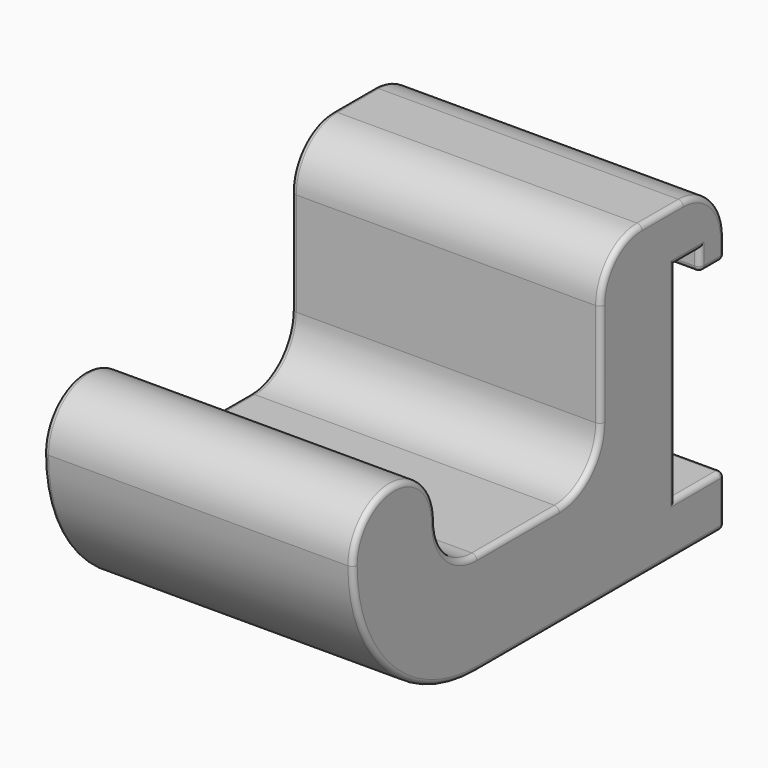
from build123d import *

# Parameters (mm, degrees)
F0_W         = 30
F0_H         = 30
F1_DEPTH     = 15
F3_DEPTH     = 30.001
F5_DEPTH     = 30
F6_R         = 5
F7_R         = 0.5
F8_T1_DEPTH  = 29
F8_S5_W      = 0.5
F8_S5_H      = 0.5
F8_T6_DEPTH  = 0.5
F8_S11_W     = 0.5
F8_S11_H     = 0.5
F8_T12_DEPTH = 0.5
F8_S17_W     = 0.5
F8_S17_H     = 0.5
F8_T18_DEPTH = 0.5
F8_S23_W     = 0.5
F8_S23_H     = 0.5
F8_T24_DEPTH = 0.5
F8_S29_W     = 0.5
F8_S29_H     = 0.5
F8_T30_DEPTH = 0.5
F8_S35_W     = 0.5
F8_S35_H     = 0.5
F8_T36_DEPTH = 0.5
F8_S41_W     = 0.5
F8_S41_H     = 0.5
F8_T42_DEPTH = 0.5
F8_S47_W     = 0.5
F8_S47_H     = 0.5
F8_T48_DEPTH = 0.5


# Not quite as in the source:
# - a fillet or chamfer that OpenCascade refuses, or shapes differently, is made with other operations: its cross-section is extruded or revolved along the edge and cut away or added


with BuildPart() as f1:
    # F0 (on Front) → F1 (new body)
    with BuildSketch(Plane.XZ):
        with Locations((15, 15)):
            Rectangle(F0_W, F0_H)
    extrude(amount=F1_DEPTH)

    # F2 (on face) → F3 (cut, through all)
    with BuildSketch(Plane.YZ.offset(30)):
        Polygon((-6, 5), (0, 5), (0, 23), (-3, 23), (-3, 25), (-6, 25), align=None)
    extrude(amount=-F3_DEPTH, mode=Mode.SUBTRACT)

    # F4 (on face) → F5 (join, through all)
    with BuildSketch(Plane.YZ.offset(30)):
        with BuildLine():
            Line((-30, 0), (-15, 0))
            Line((-15, 0), (-15, 10))
            Line((-15, 10), (-30, 10))
            ThreePointArc((-30, 10), (-33.5355339059, 11.4644660941), (-35, 15))
            ThreePointArc((-35, 15), (-40, 20), (-45, 15))
            ThreePointArc((-45, 15), (-40.6066017178, 4.3933982822), (-30, 0))
        make_face()
    extrude(amount=-F5_DEPTH)

    # F6
    f6_edges = [f1.edges().sort_by_distance(p)[0] for p in [
        (15, -15, 10),
        (15, -15, 30),
        (15, 0, 30),
    ]]
    fillet(f6_edges, radius=F6_R)

    # F7
    f7_edges = [f1.edges().sort_by_distance(p)[0] for p in [
        (30, -25, 10),
        (30, -16.464466, 11.464466),
        (30, -33.535534, 11.464466),
        (30, -15, 20),
        (30, -40, 20),
        (30, -13.535534, 28.535534),
        (30, -40.606602, 4.393398),
        (30, -7.5, 30),
        (30, -15, 0),
        (30, -1.464466, 28.535534),
        (30, 0, 2.5),
        (30, 0, 24),
        (30, -3, 5),
        (30, -1.5, 23),
        (30, -6, 15),
        (30, -3, 24),
        (30, -4.5, 25),
        (0, 0, 24),
        (0, -1.464466, 28.535534),
        (0, -1.5, 23),
        (0, -7.5, 30),
        (0, -3, 24),
        (0, -13.535534, 28.535534),
        (0, -4.5, 25),
        (0, -15, 20),
        (0, -6, 15),
        (0, -16.464466, 11.464466),
        (0, -3, 5),
        (0, -25, 10),
        (0, 0, 2.5),
        (0, -33.535534, 11.464466),
        (0, -15, 0),
        (0, -40, 20),
        (0, -40.606602, 4.393398),
    ]]
    fillet(f7_edges, radius=F7_R)

    # F8: fillet of radius 0.5 on 4 edges, made by hand

    # F8_s2 → F8_t1 (cut)
    with BuildSketch(Plane.YZ.offset(0.5)):
        with BuildLine():
            ThreePointArc((0, 4.5), (-0.1464466094, 4.8535533906), (-0.5, 5))
            Line((-0.5, 5), (0, 5))
            Line((0, 5), (0, 4.5))
        make_face()
        with BuildLine():
            ThreePointArc((-0.5, 0), (-0.1464466094, 0.1464466094), (0, 0.5))
            Line((0, 0.5), (0, 0))
            Line((0, 0), (-0.5, 0))
        make_face()
        with BuildLine():
            ThreePointArc((-0.5, 23), (-0.1464466094, 23.1464466094), (0, 23.5))
            Line((0, 23.5), (0, 23))
            Line((0, 23), (-0.5, 23))
        make_face()
        with BuildLine():
            ThreePointArc((-3, 23.5), (-2.8535533906, 23.1464466094), (-2.5, 23))
            Line((-2.5, 23), (-3, 23))
            Line((-3, 23), (-3, 23.5))
        make_face()
    extrude(amount=F8_T1_DEPTH, mode=Mode.SUBTRACT)


with BuildPart() as f8_tool4:
    # F8_s5 → F8_t6 (new body)
    with BuildSketch(Plane.XZ.offset(2.5)):
        with Locations((29.75, 23.25)):
            Rectangle(F8_S5_W, F8_S5_H)
    extrude(amount=F8_T6_DEPTH)

    # F8_s7 → F8_t8 (revolve, cut)
    with BuildSketch(Plane(origin=(29.5, -2.5, 23.5), x_dir=(-0.7071067812, 0, 0.7071067812), z_dir=(0.7071067812, 0, 0.7071067812))):
        with BuildLine():
            ThreePointArc((0, -0.5), (0.5, 0), (0, 0.5))
            Line((0, 0.5), (0, -0.5))
        make_face()
    revolve(axis=Axis((29.5, -2.5, 23.5), (0, -1, 0)), mode=Mode.SUBTRACT)


with BuildPart() as f1_1:
    add(f1.part)

    # F8_t3: cut F8_tool4
    add(f8_tool4.part, mode=Mode.SUBTRACT)


with BuildPart() as f8_tool10:
    # F8_s11 → F8_t12 (new body)
    with BuildSketch(Plane.XZ.offset(2.5)):
        with Locations((0.25, 23.25)):
            Rectangle(F8_S11_W, F8_S11_H)
    extrude(amount=F8_T12_DEPTH)

    # F8_s13 → F8_t14 (revolve, cut)
    with BuildSketch(Plane(origin=(0.5, -2.5, 23.5), x_dir=(0.7071067812, 0, 0.7071067812), z_dir=(0.7071067812, 0, -0.7071067812))):
        with BuildLine():
            ThreePointArc((0, -0.5), (0.5, 0), (0, 0.5))
            Line((0, 0.5), (0, -0.5))
        make_face()
    revolve(axis=Axis((0.5, -2.5, 23.5), (0, -1, 0)), mode=Mode.SUBTRACT)


with BuildPart() as f1_2:
    add(f1_1.part)

    # F8_t9: cut F8_tool10
    add(f8_tool10.part, mode=Mode.SUBTRACT)


with BuildPart() as f8_tool16:
    # F8_s17 → F8_t18 (new body)
    with BuildSketch(Plane.XY.offset(23.5)):
        with Locations((29.75, -0.25)):
            Rectangle(F8_S17_W, F8_S17_H)
    extrude(amount=-F8_T18_DEPTH)

    # F8_s19 → F8_t20 (revolve, cut)
    with BuildSketch(Plane(origin=(29.5, -0.5, 23.5), x_dir=(-0.7071067812, -0.7071067812, 0), z_dir=(0.7071067812, -0.7071067812, 0))):
        with BuildLine():
            ThreePointArc((0, -0.5), (0.5, 0), (0, 0.5))
            Line((0, 0.5), (0, -0.5))
        make_face()
    revolve(axis=Axis((29.5, -0.5, 23.5), (0, 0, -1)), mode=Mode.SUBTRACT)


with BuildPart() as f1_3:
    add(f1_2.part)

    # F8_t15: cut F8_tool16
    add(f8_tool16.part, mode=Mode.SUBTRACT)


with BuildPart() as f8_tool22:
    # F8_s23 → F8_t24 (new body)
    with BuildSketch(Plane.XY.offset(23.5)):
        with Locations((0.25, -0.25)):
            Rectangle(F8_S23_W, F8_S23_H)
    extrude(amount=-F8_T24_DEPTH)

    # F8_s25 → F8_t26 (revolve, cut)
    with BuildSketch(Plane(origin=(0.5, -0.5, 23.5), x_dir=(0.7071067812, -0.7071067812, 0), z_dir=(0.7071067812, 0.7071067812, 0))):
        with BuildLine():
            ThreePointArc((0, -0.5), (0.5, 0), (0, 0.5))
            Line((0, 0.5), (0, -0.5))
        make_face()
    revolve(axis=Axis((0.5, -0.5, 23.5), (0, 0, -1)), mode=Mode.SUBTRACT)


with BuildPart() as f1_4:
    add(f1_3.part)

    # F8_t21: cut F8_tool22
    add(f8_tool22.part, mode=Mode.SUBTRACT)


with BuildPart() as f8_tool28:
    # F8_s29 → F8_t30 (new body)
    with BuildSketch(Plane.XY.offset(0.5)):
        with Locations((0.25, -0.25)):
            Rectangle(F8_S29_W, F8_S29_H)
    extrude(amount=-F8_T30_DEPTH)

    # F8_s31 → F8_t32 (revolve, cut)
    with BuildSketch(Plane(origin=(0.5, -0.5, 0.5), x_dir=(0.7071067812, -0.7071067812, 0), z_dir=(0.7071067812, 0.7071067812, 0))):
        with BuildLine():
            ThreePointArc((0, -0.5), (0.5, 0), (0, 0.5))
            Line((0, 0.5), (0, -0.5))
        make_face()
    revolve(axis=Axis((0.5, -0.5, 0.5), (0, 0, -1)), mode=Mode.SUBTRACT)


with BuildPart() as f1_5:
    add(f1_4.part)

    # F8_t27: cut F8_tool28
    add(f8_tool28.part, mode=Mode.SUBTRACT)


with BuildPart() as f8_tool34:
    # F8_s35 → F8_t36 (new body)
    with BuildSketch(Plane.XY.offset(0.5)):
        with Locations((29.75, -0.25)):
            Rectangle(F8_S35_W, F8_S35_H)
    extrude(amount=-F8_T36_DEPTH)

    # F8_s37 → F8_t38 (revolve, cut)
    with BuildSketch(Plane(origin=(29.5, -0.5, 0.5), x_dir=(-0.7071067812, -0.7071067812, 0), z_dir=(0.7071067812, -0.7071067812, 0))):
        with BuildLine():
            ThreePointArc((0, -0.5), (0.5, 0), (0, 0.5))
            Line((0, 0.5), (0, -0.5))
        make_face()
    revolve(axis=Axis((29.5, -0.5, 0.5), (0, 0, -1)), mode=Mode.SUBTRACT)


with BuildPart() as f1_6:
    add(f1_5.part)

    # F8_t33: cut F8_tool34
    add(f8_tool34.part, mode=Mode.SUBTRACT)


with BuildPart() as f8_tool40:
    # F8_s41 → F8_t42 (new body)
    with BuildSketch(Plane.XZ.offset(0.5)):
        with Locations((29.75, 4.75)):
            Rectangle(F8_S41_W, F8_S41_H)
    extrude(amount=-F8_T42_DEPTH)

    # F8_s43 → F8_t44 (revolve, cut)
    with BuildSketch(Plane(origin=(29.5, -0.5, 4.5), x_dir=(-0.7071067812, 0, -0.7071067812), z_dir=(0.7071067812, 0, -0.7071067812))):
        with BuildLine():
            ThreePointArc((0, -0.5), (0.5, 0), (0, 0.5))
            Line((0, 0.5), (0, -0.5))
        make_face()
    revolve(axis=Axis((29.5, -0.5, 4.5), (0, 1, 0)), mode=Mode.SUBTRACT)


with BuildPart() as f1_7:
    add(f1_6.part)

    # F8_t39: cut F8_tool40
    add(f8_tool40.part, mode=Mode.SUBTRACT)


with BuildPart() as f8_tool46:
    # F8_s47 → F8_t48 (new body)
    with BuildSketch(Plane.XZ.offset(0.5)):
        with Locations((0.25, 4.75)):
            Rectangle(F8_S47_W, F8_S47_H)
    extrude(amount=-F8_T48_DEPTH)

    # F8_s49 → F8_t50 (revolve, cut)
    with BuildSketch(Plane(origin=(0.5, -0.5, 4.5), x_dir=(0.7071067812, 0, -0.7071067812), z_dir=(0.7071067812, 0, 0.7071067812))):
        with BuildLine():
            ThreePointArc((0, -0.5), (0.5, 0), (0, 0.5))
            Line((0, 0.5), (0, -0.5))
        make_face()
    revolve(axis=Axis((0.5, -0.5, 4.5), (0, 1, 0)), mode=Mode.SUBTRACT)


with BuildPart() as f1_8:
    add(f1_7.part)

    # F8_t45: cut F8_tool46
    add(f8_tool46.part, mode=Mode.SUBTRACT)


solid = f1_8.part
